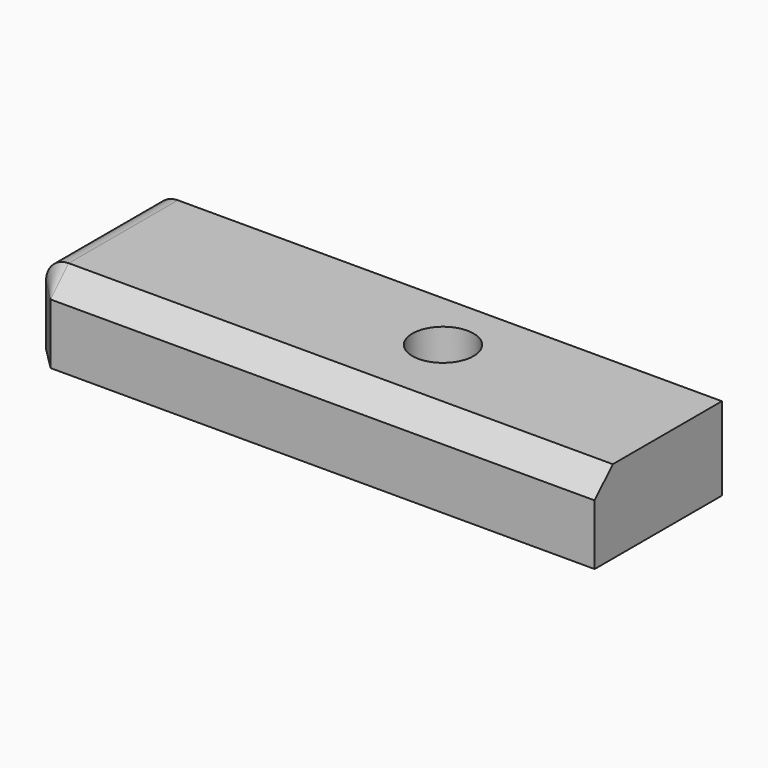
from build123d import *

# Parameters (mm, degrees)
F0_W     = 35.6490109116
F0_H     = 18.6256058514
F1_DEPTH = 127
F2_R     = 6.8542963407
F3_DEPTH = 25.4
F4_R     = 5.08
F5_SIZE  = 5.07999


# Not quite as in the source:
# - a fillet or chamfer is up to 0.001 mm smaller than in the source, because OpenCascade refuses the exact size


with BuildPart() as f1:
    # F0 (on Right) → F1 (new body)
    with BuildSketch(Plane.YZ):
        with Locations((-41.2567211315, -34.4473589212)):
            Rectangle(F0_W, F0_H)
    extrude(amount=F1_DEPTH)

    # F2 (on face) → F3 (cut)
    with BuildSketch(Plane.XY.offset(-25.1345559955)):
        with Locations((75.5256735351, -37.2293450889)):
            Circle(F2_R)
    extrude(amount=-F3_DEPTH, mode=Mode.SUBTRACT)

    # F4
    f4_edges = [f1.edges().sort_by_distance(p)[0] for p in [
        (0, -41.256721, -25.134556),
    ]]
    fillet(f4_edges, radius=F4_R)

    # F5 (size 5.08 in the source; OpenCascade refuses exactly that, so slightly less here)
    f5_edges = [f1.edges().sort_by_distance(p)[0] for p in [
        (66.04, -59.081227, -25.134556),
    ]]
    chamfer(f5_edges, length=F5_SIZE)


solid = f1.part
